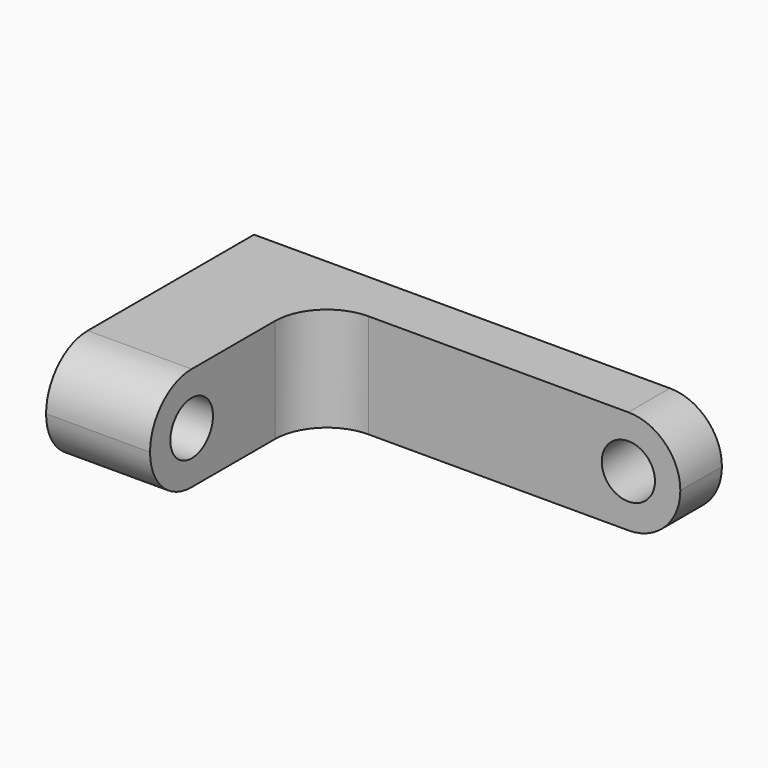
from build123d import *

# Parameters (mm, degrees)
F1_DEPTH = 6.35
F2_R     = 3.17499
F3_R     = 1.6256
F4_DEPTH = 6.351
F5_R     = 1.6256
F6_DEPTH = 3.176


# Not quite as in the source:
# - a fillet or chamfer is up to 0.001 mm smaller than in the source, because OpenCascade refuses the exact size


with BuildPart() as f1:
    # F0 (on Top) → F1 (new body)
    with BuildSketch(Plane.XY):
        Polygon((0, 0), (0, -15.875), (6.35, -15.875), (6.35, -3.175), (28.575, -3.175), (28.575, 0), align=None)
    extrude(amount=F1_DEPTH)

    # F2 (radius 3.175 in the source; OpenCascade refuses exactly that, so slightly less here)
    f2_edges = [f1.edges().sort_by_distance(p)[0] for p in [
        (3.175, -15.875, 6.35),
        (3.175, -15.875, 0),
        (28.575, -1.5875, 6.35),
        (28.575, -1.5875, 0),
        (6.35, -3.175, 3.175),
    ]]
    fillet(f2_edges, radius=F2_R)

    # F3 (on face) → F4 (cut, through all)
    with BuildSketch(Plane.YZ.offset(6.35)):
        with Locations((-12.7, 3.175)):
            Circle(F3_R)
    extrude(amount=-F4_DEPTH, mode=Mode.SUBTRACT)

    # F5 (on face) → F6 (cut, through all)
    with BuildSketch(Plane.XZ.offset(3.175)):
        with Locations((25.4, 3.175)):
            Circle(F5_R)
    extrude(amount=-F6_DEPTH, mode=Mode.SUBTRACT)


solid = f1.part
